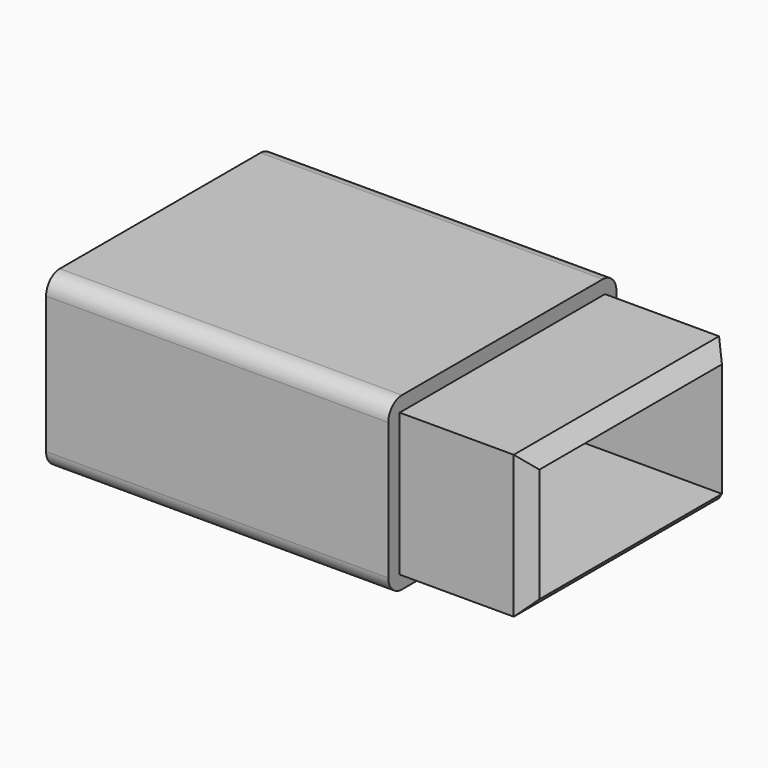
from build123d import *

# Parameters (mm, degrees)
F0_W        = 49.9999988824
F0_H        = 29.9999988824
F0_W_2      = 45.0000008941
F0_H_2      = 25.0000008941
F0_W_3      = 40
F0_H_3      = 20
F1_DEPTH    = 60
F2_DEPTH    = 55
F3_DEPTH    = 25
F4_T1_DEPTH = 50.7168307737
F4_T3_DEPTH = 70.7168307737
F5_R        = 3
F7_DEPTH    = 2


# Not quite as in the source:
# - a fillet or chamfer that OpenCascade refuses, or shapes differently, is made with other operations: its cross-section is extruded or revolved along the edge and cut away or added


with BuildPart() as f1:
    # F0 (on Right) → F1 (new body)
    with BuildSketch(Plane.YZ):
        with Locations((10.3521584719, 3.6993094161)):
            Rectangle(F0_W, F0_H)
        with Locations((10.3521584719, 3.6993094161)):
            Rectangle(F0_W_2, F0_H_2, mode=Mode.SUBTRACT)
        with Locations((10.3521584719, 3.6993094161)):
            Rectangle(F0_W_2, F0_H_2)
        with Locations((10.3521584719, 3.6993094161)):
            Rectangle(F0_W_3, F0_H_3, mode=Mode.SUBTRACT)
        with Locations((10.3521584719, 3.6993094161)):
            Rectangle(F0_W_3, F0_H_3)
    extrude(amount=-F1_DEPTH)

    # F0 (on Right) → F2 (cut)
    with BuildSketch(Plane.YZ):
        with Locations((10.3521584719, 3.6993094161)):
            Rectangle(F0_W_3, F0_H_3)
    extrude(amount=-F2_DEPTH, mode=Mode.SUBTRACT)

    # F0 (on Right) → F3 (join)
    with BuildSketch(Plane.YZ):
        with Locations((10.3521584719, 3.6993094161)):
            Rectangle(F0_W_2, F0_H_2)
        with Locations((10.3521584719, 3.6993094161)):
            Rectangle(F0_W_3, F0_H_3, mode=Mode.SUBTRACT)
    extrude(amount=F3_DEPTH)

    # F4: chamfer of 5 on 4 edges, made by hand

    # F4_s2 → F4_t1 (cut)
    with BuildSketch(Plane.XY.offset(-21.6591059707)):
        Polygon((25, -7.1478419751), (20, -12.1478419751), (25, -12.1478419751), align=None)
        Polygon((25, 27.852158919), (20, 32.852158919), (25, 32.852158919), align=None)
    extrude(amount=F4_T1_DEPTH, mode=Mode.SUBTRACT)

    # F4_s4 → F4_t3 (cut)
    with BuildSketch(Plane.XZ.offset(-45.7105738588)):
        Polygon((20, -8.8006910309), (25, -3.8006910309), (25, -8.8006910309), align=None)
        Polygon((25, 11.1993098632), (20, 16.1993098632), (25, 16.1993098632), align=None)
    extrude(amount=F4_T3_DEPTH, mode=Mode.SUBTRACT)

    # F5
    f5_edges = [f1.edges().sort_by_distance(p)[0] for p in [
        (-30, 35.352158, -11.30069),
        (-30, 35.352158, 18.699309),
        (-30, -14.647841, -11.30069),
        (-30, -14.647841, 18.699309),
    ]]
    fillet(f5_edges, radius=F5_R)

    # F6 (on face) → F7 (cut)
    with BuildSketch(Plane(origin=(0, 0, -11.3006900251), x_dir=(1, 0, 0), z_dir=(0, 0, -1))):
        with BuildLine():
            Line((-40.5811635508, -19.8521577269), (-36.5980909465, -19.8521577269))
            Line((-36.5980909465, -19.8521577269), (-36.5980909465, -1.0129664961))
            Line((-36.5980909465, -1.0129664961), (-39.8719622175, -1.0129664961))
            Line((-39.8719622175, -1.0129664961), (-45.941406186, -5.8454313948))
            Line((-45.941406186, -5.8454313948), (-44.0199653644, -8.2410475264))
            Line((-44.0199653644, -8.2410475264), (-41.8552519925, -6.5010303018))
            add(Edge.make_bspline(
                [(-40.4780819617, -5.2022022786), (-41.4676652174, -6.1917855343), (-41.8552519925, -6.5010303018)],
                knots=[0, 0, 0, 1, 1, 1], degree=2))
            Line((-40.4780819617, -5.2022022786), (-40.5399309151, -7.1607524722))
            Line((-40.5399309151, -7.1607524722), (-40.5811635508, -8.9502488597))
            Line((-40.5811635508, -8.9502488597), (-40.5811635508, -19.8521577269))
        make_face()
        with BuildLine():
            Line((-26.8667704258, -19.8521577269), (-22.8777154217, -19.8521577269))
            add(Edge.make_bspline(
                [(-19.9318596147, -17.7389851496), (-21.0133994036, -19.326806957), (-22.8777154217, -19.8521577269)],
                knots=[0, 0, 0, 0.6691374514, 0.6691374514, 0.6691374514], degree=2))
            add(Edge.make_bspline(
                [(-18.315540297, -10.4346237433), (-18.315540297, -15.3660469676), (-19.9318596147, -17.7389851496)],
                knots=[0, 0, 0, 1, 1, 1], degree=2))
            add(Edge.make_bspline(
                [(-19.9834004093, -3.1900496586), (-18.315540297, -5.664007798), (-18.315540297, -10.4346237433)],
                knots=[0, 0, 0, 1, 1, 1], degree=2))
            add(Edge.make_bspline(
                [(-23.4706324827, -0.852159217), (-21.2601126538, -1.2962861316), (-19.9834004093, -3.1900496586)],
                knots=[0.234520788, 0.234520788, 0.234520788, 1, 1, 1], degree=2))
            Line((-23.4706324827, -0.852159217), (-26.4191418917, -0.852159217))
            add(Edge.make_bspline(
                [(-29.8730480712, -3.0807831742), (-28.6475822393, -1.2833288146), (-26.4191418917, -0.852159217)],
                knots=[0, 0, 0, 0.7601220886, 0.7601220886, 0.7601220886], degree=2))
            add(Edge.make_bspline(
                [(-31.4852441253, -10.4346237433), (-31.4852441253, -5.445474829), (-29.8730480712, -3.0807831742)],
                knots=[0, 0, 0, 1, 1, 1], degree=2))
            add(Edge.make_bspline(
                [(-29.8297538037, -17.6627047736), (-31.4852441253, -15.2134862157), (-31.4852441253, -10.4346237433)],
                knots=[0, 0, 0, 1, 1, 1], degree=2))
            add(Edge.make_bspline(
                [(-26.8667704258, -19.8521577269), (-28.7134061438, -19.3142876129), (-29.8297538037, -17.6627047736)],
                knots=[0.3256694736, 0.3256694736, 0.3256694736, 1, 1, 1], degree=2))
        make_face()
        with BuildLine():
            add(Edge.make_bspline(
                [(-27.5269111024, -10.4346237433), (-27.5269111024, -13.8981651383), (-26.9290378854, -15.3990330761)],
                knots=[0, 0, 0, 1, 1, 1], degree=2))
            add(Edge.make_bspline(
                [(-26.92285299, -5.4537213561), (-27.5269111024, -6.9669590847), (-27.5269111024, -10.4346237433)],
                knots=[0, 0, 0, 1, 1, 1], degree=2))
            add(Edge.make_bspline(
                [(-24.9127620019, -3.9404836276), (-26.3187948777, -3.9404836276), (-26.92285299, -5.4537213561)],
                knots=[0, 0, 0, 1, 1, 1], degree=2))
            add(Edge.make_bspline(
                [(-22.908855909, -5.4537213561), (-23.535591971, -3.9404836276), (-24.9127620019, -3.9404836276)],
                knots=[0, 0, 0, 1, 1, 1], degree=2))
            add(Edge.make_bspline(
                [(-22.2821198471, -10.4346237433), (-22.2821198471, -6.9669590847), (-22.908855909, -5.4537213561)],
                knots=[0, 0, 0, 1, 1, 1], degree=2))
            add(Edge.make_bspline(
                [(-22.9006093819, -15.3804783901), (-22.2821198471, -13.8610557662), (-22.2821198471, -10.4346237433)],
                knots=[0, 0, 0, 1, 1, 1], degree=2))
            add(Edge.make_bspline(
                [(-24.9127620019, -16.899901014), (-23.5190989167, -16.899901014), (-22.9006093819, -15.3804783901)],
                knots=[0, 0, 0, 1, 1, 1], degree=2))
            add(Edge.make_bspline(
                [(-26.9290378854, -15.3990330761), (-26.3311646684, -16.899901014), (-24.9127620019, -16.899901014)],
                knots=[0, 0, 0, 1, 1, 1], degree=2))
        make_face(mode=Mode.SUBTRACT)
    extrude(amount=-F7_DEPTH, mode=Mode.SUBTRACT)


solid = f1.part
